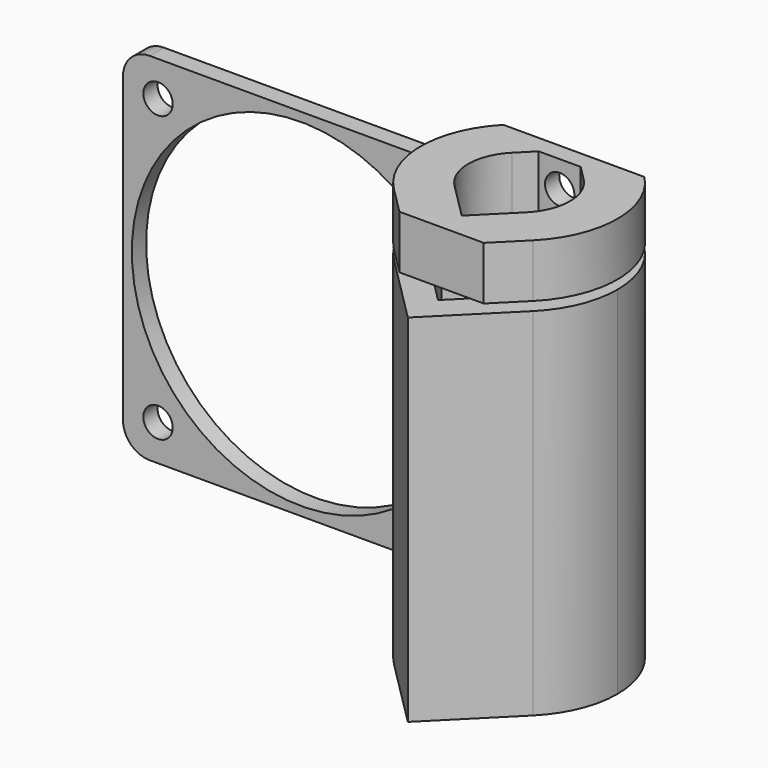
from build123d import *

# Parameters (mm, degrees)
F0_W      = 40
F0_H      = 40
F0_R      = 19
F1_DEPTH  = 2
F2_D      = 3.3
F4_DEPTH  = 20
F5_R      = 8.04999
F6_R      = 11.04999
F8_DEPTH  = 21
F9_R      = 7.55
F10_R     = 5.69999
F12_DEPTH = 6
F13_R     = 1.65
F14_DEPTH = 5
F15_R     = 3


# Not quite as in the source:
# - a fillet or chamfer is up to 0.001 mm smaller than in the source, because OpenCascade refuses the exact size


with BuildPart() as f1:
    # F0 (on Front) → F1 (new body)
    with BuildSketch(Plane.XZ):
        Rectangle(F0_W, F0_H)
        Circle(F0_R, mode=Mode.SUBTRACT)
    extrude(amount=F1_DEPTH)

    # F2 (through all)
    with Locations(Plane(origin=(0, 0, 0), x_dir=(1, 0, 0), z_dir=(0, 1, 0))):
        with Locations((-16.059378162, -16.059378162), (15.940621838, -16.059378162), (15.940621838, 15.940621838), (-16.059378162, 15.940621838)):
            Hole(F2_D / 2)

    # F3 (on Top) → F4 (join, symmetric)
    with BuildSketch(Plane.XY):
        Polygon((20.7, -15.6270598642), (27.1729401358, -22.1), (31.75, -26.6770598642), (36.3270598642, -22.1), (42.8, -15.6270598642), (42.8, -6.4729401358), (36.3270598642, 0), (27.1729401358, 0), (20, 0), (20, -2), (20.7, -2), (20.7, -6.4729401358), align=None)
        Polygon((39.8, -7.7155808229), (39.8, -14.3844191771), (35.0844191771, -19.1), (31.75, -22.4344191771), (28.4155808229, -19.1), (23.7, -14.3844191771), (23.7, -7.7155808229), (28.4155808229, -3), (35.0844191771, -3), align=None, mode=Mode.SUBTRACT)
    extrude(amount=F4_DEPTH, both=True)

    # F5 (radius 8.05 in the source; OpenCascade refuses exactly that, so slightly less here)
    f5_edges = [f1.edges().sort_by_distance(p)[0] for p in [
        (23.7, -7.715581, 0),
        (23.7, -14.384419, 0),
        (39.8, -7.715581, 0),
        (39.8, -14.384419, 0),
    ]]
    fillet(f5_edges, radius=F5_R)

    # F6 (radius 11.05 in the source; OpenCascade refuses exactly that, so slightly less here)
    f6_edges = [f1.edges().sort_by_distance(p)[0] for p in [
        (20.7, -15.62706, 0),
        (42.8, -15.62706, 0),
        (42.8, -6.47294, 0),
    ]]
    fillet(f6_edges, radius=F6_R)

    # F15
    f15_edges = [f1.edges().sort_by_distance(p)[0] for p in [
        (-20, -1, 20),
        (-20, -1, -20),
    ]]
    fillet(f15_edges, radius=F15_R)


with BuildPart() as f8:
    # F7 (on Top) → F8 (new body, symmetric)
    with BuildSketch(Plane.XY):
        Polygon((24.05, -7.8605555697), (24.05, -14.2394444303), (31.75, -21.9394444303), (39.45, -14.2394444303), (39.45, -7.8605555697), (34.9394444303, -3.35), (28.5605555697, -3.35), align=None)
        Polygon((31.75, -19.1110173055), (26.05, -13.4110173055), (26.05, -8.6889826945), (29.3889826945, -5.35), (34.1110173055, -5.35), (37.45, -8.6889826945), (37.45, -13.4110173055), align=None, mode=Mode.SUBTRACT)
    extrude(amount=F8_DEPTH, both=True)

    # F9
    f9_edges = [f8.edges().sort_by_distance(p)[0] for p in [
        (39.45, -14.239444, 0),
        (39.45, -7.860556, 0),
        (24.05, -14.239444, 0),
        (24.05, -7.860556, 0),
    ]]
    fillet(f9_edges, radius=F9_R)

    # F10 (radius 5.7 in the source; OpenCascade refuses exactly that, so slightly less here)
    f10_edges = [f8.edges().sort_by_distance(p)[0] for p in [
        (37.45, -8.688983, 0),
        (37.45, -13.411017, 0),
        (26.05, -8.688983, 0),
        (26.05, -13.411017, 0),
    ]]
    fillet(f10_edges, radius=F10_R)

    # F11 (on face) → F12 (join)
    with BuildSketch(Plane.XY.offset(21)):
        with BuildLine():
            ThreePointArc((23.8245662579, -3.35), (20.7002874642, -11.1297049374), (23.9364700679, -18.8635299321))
            Line((23.9364700679, -18.8635299321), (27.0123845661, -21.9394444303))
            Line((27.0123845661, -21.9394444303), (36.4876154339, -21.9394444303))
            Line((36.4876154339, -21.9394444303), (39.5635299321, -18.8635299321))
            ThreePointArc((39.5635299321, -18.8635299321), (42.7997125358, -11.1297049374), (39.6754337421, -3.35))
            Line((39.6754337421, -3.35), (23.8245662579, -3.35))
        make_face()
        with BuildLine():
            Line((27.7194913472, -7.0194913472), (29.3889826945, -5.35))
            Line((29.3889826945, -5.35), (34.1110173055, -5.35))
            Line((34.1110173055, -5.35), (35.7805086528, -7.0194913472))
            ThreePointArc((35.7805086528, -7.0194913472), (37.45, -11.05), (35.7805086528, -15.0805086528))
            Line((35.7805086528, -15.0805086528), (31.75, -19.1110173055))
            Line((31.75, -19.1110173055), (27.7194913472, -15.0805086528))
            ThreePointArc((27.7194913472, -15.0805086528), (26.05, -11.05), (27.7194913472, -7.0194913472))
        make_face(mode=Mode.SUBTRACT)
    extrude(amount=F12_DEPTH)

    # F13 (on face) → F14 (cut)
    with BuildSketch(Plane(origin=(0, -3.35, 0), x_dir=(-1, 0, 0), z_dir=(0, 1, 0))):
        with Locations((-31.75, 24)):
            Circle(F13_R)
    extrude(amount=-F14_DEPTH, mode=Mode.SUBTRACT)


solid = Compound([f1.part, f8.part])
